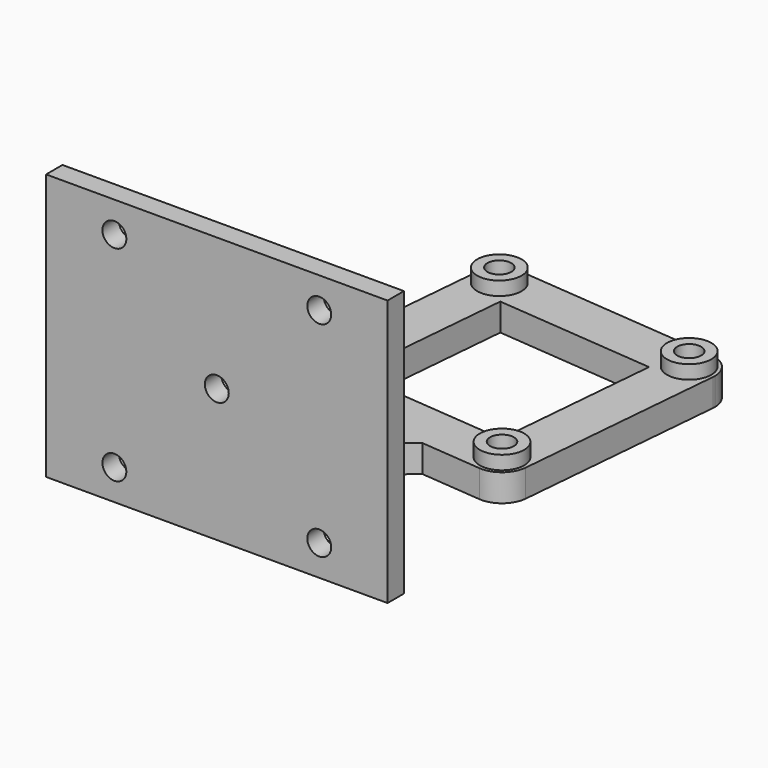
from build123d import *

# Parameters (mm, degrees)
F0_R         = 1.75
F1_DEPTH     = 4
F2_W         = 50
F2_H         = 3
F3_DEPTH     = 35
F4_R         = 1.75
F5_DEPTH     = 3
F6_T1_DEPTH  = 4
F6_T6_DEPTH  = 28.6040226041
F6_T13_DEPTH = 28.6040226041
F6_S15_R     = 1.75
F6_T16_DEPTH = 16
F6_T19_DEPTH = 15.1872089077
F6_T26_DEPTH = 13.4620824192
F6_T30_DEPTH = 28.6040226041
F6_S32_R     = 1.75
F6_T33_DEPTH = 16
F7_R         = 3.25
F7_R_2       = 1.75
F8_DEPTH     = 2
F9_SIZE      = 2


# Not quite as in the source:
# - a fillet or chamfer that OpenCascade refuses, or shapes differently, is made with other operations: its cross-section is extruded or revolved along the edge and cut away or added


with BuildPart() as f1:
    # F0 (on Top) → F1 (new body)
    with BuildSketch(Plane.XY):
        Polygon((-4.0152793502, 1.5), (-25, 1.5), (-25, -1.5), (25, -1.5), (25, 1.5), (4.0152793502, 1.5), align=None)
        Polygon((-1.8013300137, 26.8055567119), (-4.0152793502, 1.5), (4.0152793502, 1.5), (6.1682275711, 26.10831077), align=None)
        with BuildLine():
            Line((-12.7594716927, 27.7642698822), (-1.8013300137, 26.8055567119))
            Line((-1.8013300137, 26.8055567119), (-1.4744959784, 30.5412868298))
            Line((-1.4744959784, 30.5412868298), (6.4950616064, 29.8440408878))
            Line((6.4950616064, 29.8440408878), (6.1682275711, 26.10831077))
            Line((6.1682275711, 26.10831077), (17.1263692501, 25.1495975997))
            ThreePointArc((17.1263692501, 25.1495975997), (14.9197400068, 31.6501177306), (21.2032032854, 28.8853277176))
            ThreePointArc((21.2032032854, 28.8853277176), (21.1996341163, 28.721755015), (21.1889334032, 28.5584936823))
            Line((21.1889334032, 28.5584936823), (23.8907614284, 59.4405293231))
            ThreePointArc((23.8907614284, 59.4405293231), (17.2823646489, 57.3569098221), (20.4818653459, 63.5030934763))
            Line((20.4818653459, 63.5030934763), (-9.4039755969, 66.1177657587))
            ThreePointArc((-9.4039755969, 66.1177657587), (-6.9660196192, 64.9154989194), (-5.9808096322, 62.3820356408))
            ThreePointArc((-5.9808096322, 62.3820356408), (-9.8943823348, 58.6356048099), (-13.46653975, 62.7088696761))
            Line((-13.46653975, 62.7088696761), (-16.1683677752, 31.8268340353))
            ThreePointArc((-16.1683677752, 31.8268340353), (-12.2690649548, 35.2464308309), (-8.6826376574, 31.5))
            ThreePointArc((-8.6826376574, 31.5), (-9.8991743788, 28.735209987), (-12.7594716927, 27.7642698822))
        make_face()
        Polygon((-8.9117487246, 34.4543766049), (-6.7764330273, 58.8611467081), (16.6341423778, 56.8129867535), (14.4988266805, 32.4062166503), align=None, mode=Mode.SUBTRACT)
        Polygon((-1.4744959784, 30.5412868298), (-1.8013300137, 26.8055567119), (6.1682275711, 26.10831077), (6.4950616064, 29.8440408878), align=None)
        with BuildLine():
            ThreePointArc((-16.1683677752, 31.8268340353), (-15.3053043191, 29.0895464637), (-12.7594716927, 27.7642698822))
            ThreePointArc((-12.7594716927, 27.7642698822), (-9.8991743788, 28.735209987), (-8.6826376574, 31.5))
            ThreePointArc((-8.6826376574, 31.5), (-12.2690649548, 35.2464308309), (-16.1683677752, 31.8268340353))
        make_face()
        with Locations((-12.4326376574, 31.5)):
            Circle(F0_R, mode=Mode.SUBTRACT)
        with BuildLine():
            ThreePointArc((21.2032032854, 28.8853277176), (14.9197400068, 31.6501177306), (17.1263692501, 25.1495975997))
            ThreePointArc((17.1263692501, 25.1495975997), (19.8636568217, 26.0126610559), (21.1889334032, 28.5584936823))
            ThreePointArc((21.1889334032, 28.5584936823), (21.1996341163, 28.721755015), (21.2032032854, 28.8853277176))
        make_face()
        with Locations((17.4532032854, 28.8853277176)):
            Circle(F0_R, mode=Mode.SUBTRACT)
        with BuildLine():
            ThreePointArc((-9.4039755969, 66.1177657587), (-12.1412631685, 65.2547023025), (-13.46653975, 62.7088696761))
            ThreePointArc((-13.46653975, 62.7088696761), (-9.8943823348, 58.6356048099), (-5.9808096322, 62.3820356408))
            ThreePointArc((-5.9808096322, 62.3820356408), (-6.9660196192, 64.9154989194), (-9.4039755969, 66.1177657587))
        make_face()
        with Locations((-9.7308096322, 62.3820356408)):
            Circle(F0_R, mode=Mode.SUBTRACT)
        with BuildLine():
            ThreePointArc((20.4818653459, 63.5030934763), (17.2823646489, 57.3569098221), (23.8907614284, 59.4405293231))
            ThreePointArc((23.8907614284, 59.4405293231), (23.9014621415, 59.6037906558), (23.9050313106, 59.7673633584))
            ThreePointArc((23.9050313106, 59.7673633584), (22.9198213236, 62.300826637), (20.4818653459, 63.5030934763))
        make_face()
        with Locations((20.1550313106, 59.7673633584)):
            Circle(F0_R, mode=Mode.SUBTRACT)
    extrude(amount=F1_DEPTH)

    # F2 (on face) → F3 (join)
    with BuildSketch(Plane.XY.offset(4)):
        Rectangle(F2_W, F2_H)
    extrude(amount=F3_DEPTH)

    # F4 (on face) → F5 (cut, through all)
    with BuildSketch(Plane.XZ.offset(1.5)):
        with Locations((-15, 34.5)):
            Circle(F4_R)
        with Locations((15, 34.5)):
            Circle(F4_R)
        with Locations((-15, 4.5)):
            Circle(F4_R)
        with Locations((15, 4.5)):
            Circle(F4_R)
        with Locations((0, 19.5)):
            Circle(F4_R)
    extrude(amount=-F5_DEPTH, mode=Mode.SUBTRACT)

    # F6: chamfer of 4 on 3 edges, made by hand

    # F6_s2 → F6_t1 (join)
    with BuildSketch(Plane.XY):
        Polygon((-7.6806040462, 1.5), (-3.6958252539, 5.151377029), (-4.0152793502, 1.5), align=None)
        Polygon((8.3805133545, 1.5), (4.3957345621, 5.848622971), (4.0152793502, 1.5), align=None)
    extrude(amount=F6_T1_DEPTH)


with BuildPart() as f6_tool4:
    # F6_s5 → F6_t6 (new body)
    with BuildSketch(Plane.YZ.offset(14.302011302)):
        Polygon((1.5, 8), (5.5, 4), (1.5, 4), align=None)
    extrude(amount=-F6_T6_DEPTH)

    split(bisect_by=Plane(origin=(-4.1150149256, 0.3600171562, 0), x_dir=(0, 0, 1), z_dir=(0.9961946981, -0.0871557427, 0)), keep=Keep.TOP)

    split(bisect_by=Plane(origin=(3.8545426591, -0.3372287857, 0), x_dir=(0, 0, 1), z_dir=(-0.9961946981, 0.0871557427, 0)), keep=Keep.TOP)


with BuildPart() as f1_1:
    add(f1.part)

    # F6_t3: union F6_tool4
    add(f6_tool4.part)


with BuildPart() as f6_tool11:
    # F6_s12 → F6_t13 (new body)
    with BuildSketch(Plane.YZ.offset(14.302011302)):
        Polygon((1.5, 8), (5.5, 4), (1.5, 4), align=None)
    extrude(amount=-F6_T13_DEPTH)

    split(bisect_by=Plane(origin=(3.8545426591, -0.3372287857, 0), x_dir=(0, 0, 1), z_dir=(0.9961946981, -0.0871557427, 0)), keep=Keep.TOP)

    # F6_s15 → F6_t16 (cut, symmetric)
    with BuildSketch(Plane.XZ.offset(-3.5)):
        with Locations((15, 4.5)):
            Circle(F6_S15_R)
    extrude(amount=F6_T16_DEPTH, both=True, mode=Mode.SUBTRACT)


with BuildPart() as f6_tool17:
    # F6_s18 → F6_t19 (new body)
    with BuildSketch(Plane.XY):
        Polygon((8.3805133545, 1.5), (4.3957345621, 5.848622971), (4.0152793502, 1.5), align=None)
    extrude(amount=F6_T19_DEPTH)

    split(bisect_by=Plane.XY.offset(4), keep=Keep.TOP)


with BuildPart() as f6_tool11_1:
    add(f6_tool11.part)

    # F6_t21: intersect F6_tool17
    add(f6_tool17.part, mode=Mode.INTERSECT)


with BuildPart() as f1_2:
    add(f1_1.part)

    # F6_t9: union F6_tool11
    add(f6_tool11_1.part)


with BuildPart() as f6_tool24:
    # F6_s25 → F6_t26 (new body)
    with BuildSketch(Plane.XY):
        Polygon((-7.6806040462, 1.5), (-3.6958252539, 5.151377029), (-4.0152793502, 1.5), align=None)
    extrude(amount=F6_T26_DEPTH)

    split(bisect_by=Plane.XY.offset(4), keep=Keep.TOP)


with BuildPart() as f6_tool28:
    # F6_s29 → F6_t30 (new body)
    with BuildSketch(Plane.YZ.offset(14.302011302)):
        Polygon((1.5, 8), (5.5, 4), (1.5, 4), align=None)
    extrude(amount=-F6_T30_DEPTH)

    split(bisect_by=Plane(origin=(-4.1150149256, 0.3600171562, 0), x_dir=(0, 0, 1), z_dir=(-0.9961946981, 0.0871557427, 0)), keep=Keep.TOP)

    # F6_s32 → F6_t33 (cut, symmetric)
    with BuildSketch(Plane.XZ.offset(-3.5)):
        with Locations((-15, 4.5)):
            Circle(F6_S32_R)
    extrude(amount=F6_T33_DEPTH, both=True, mode=Mode.SUBTRACT)


with BuildPart() as f6_tool24_1:
    add(f6_tool24.part)

    # F6_t34: intersect F6_tool28
    add(f6_tool28.part, mode=Mode.INTERSECT)


with BuildPart() as f1_3:
    add(f1_2.part)

    # F6_t22: union F6_tool24
    add(f6_tool24_1.part)

    # F7 (on face) → F8 (join)
    with BuildSketch(Plane.XY.offset(4)):
        with Locations((-9.7308096322, 62.3820356408)):
            Circle(F7_R)
        with Locations((-9.7308096322, 62.3820356408)):
            Circle(F7_R_2, mode=Mode.SUBTRACT)
        with Locations((20.1550313106, 59.7673633584)):
            Circle(F7_R)
        with Locations((20.1550313106, 59.7673633584)):
            Circle(F7_R_2, mode=Mode.SUBTRACT)
        with Locations((17.4532032854, 28.8853277176)):
            Circle(F7_R)
        with Locations((17.4532032854, 28.8853277176)):
            Circle(F7_R_2, mode=Mode.SUBTRACT)
        with Locations((-12.4326376574, 31.5)):
            Circle(F7_R)
        with Locations((-12.4326376574, 31.5)):
            Circle(F7_R_2, mode=Mode.SUBTRACT)
    extrude(amount=F8_DEPTH)

    # F9
    f9_edges = [f1_3.edges().sort_by_distance(p)[0] for p in [
        (6.168228, 26.108311, 2),
        (-1.80133, 26.805557, 2),
    ]]
    chamfer(f9_edges, length=F9_SIZE)


solid = f1_3.part
